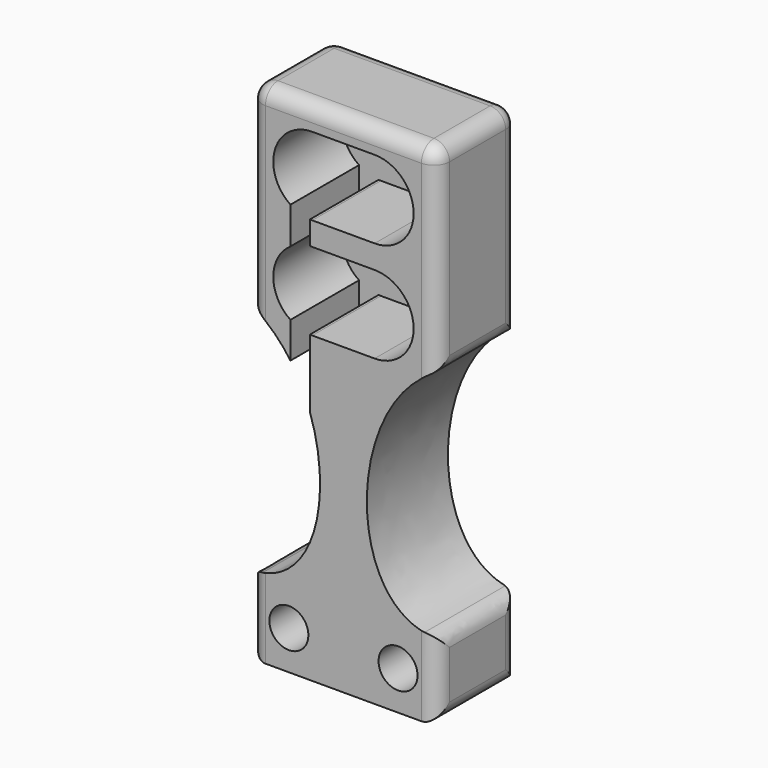
from build123d import *

# Parameters (mm, degrees)
F0_R     = 3.175
F1_DEPTH = 16.51
F2_DEPTH = 2.54
F3_R     = 2.54


# Not quite as in the source:
# - a feature names something its author has since deleted; it is built from what else it names


with BuildPart() as f1:
    # F0 (on Front) → F1 (new body)
    with BuildSketch(Plane.XZ):
        with BuildLine():
            Line((15.24, 10.16), (0, 10.16))
            Line((0, 10.16), (-15.24, 10.16))
            Line((-15.24, 10.16), (-15.24, -21.59))
            add(Edge.make_bspline(
                [(-15.24, -21.59), (-12.5713715272, -23.0241692542), (-10.3700381938, -25.1273333514), (-8.636, -27.620696738)],
                knots=[0, 0, 0, 0, 6.6715711821, 6.6715711821, 6.6715711821, 6.6715711821], degree=3))
            Line((-8.636, -27.620696738), (-8.636, -21.770928055))
            ThreePointArc((-8.636, -21.770928055), (-11.43, -16.51), (-8.636, -11.249071945))
            Line((-8.636, -11.249071945), (-8.636, -5.260928055))
            ThreePointArc((-8.636, -5.260928055), (-11.1516304709, 1.8595169871), (-5.08, 6.35))
            Line((-5.08, 6.35), (5.08, 6.35))
            ThreePointArc((5.08, 6.35), (9.5701280605, 4.4901280605), (11.43, 0))
            ThreePointArc((11.43, 0), (9.5701280605, -4.4901280605), (5.08, -6.35))
            Line((5.08, -6.35), (-5.08, -6.35))
            ThreePointArc((-5.08, -6.35), (-5.2705858603, -6.3471392792), (-5.461, -6.3385596944))
            Line((-5.461, -6.3385596944), (-5.461, -10.1714403056))
            ThreePointArc((-5.461, -10.1714403056), (-5.2705858603, -10.1628607208), (-5.08, -10.16))
            Line((-5.08, -10.16), (5.08, -10.16))
            ThreePointArc((5.08, -10.16), (9.5701280605, -12.0198719395), (11.43, -16.51))
            ThreePointArc((11.43, -16.51), (9.5701280605, -21.0001280605), (5.08, -22.86))
            Line((5.08, -22.86), (-5.08, -22.86))
            ThreePointArc((-5.08, -22.86), (-5.2705858603, -22.8571392792), (-5.461, -22.8485596944))
            Line((-5.461, -22.8485596944), (-5.461, -33.9487214282))
            add(Edge.make_bspline(
                [(-5.461, -33.9487214282), (-1.4642877536, -45.4909328609), (-4.7239544203, -59.7580237479), (-15.24, -59.69)],
                knots=[11.8098860506, 11.8098860506, 11.8098860506, 11.8098860506, 38.1, 38.1, 38.1, 38.1], degree=3))
            Line((-15.24, -59.69), (-15.24, -72.39))
            Line((-15.24, -72.39), (15.24, -72.39))
            Line((15.24, -72.39), (15.24, -59.69))
            add(Edge.make_bspline(
                [(15.24, -21.59), (0, -29.7802519053), (0, -59.7885809647), (15.24, -59.69)],
                knots=[0, 0, 0, 0, 38.1, 38.1, 38.1, 38.1], degree=3))
            Line((15.24, -21.59), (15.24, 10.16))
        make_face()
        with Locations((-8.89, -66.04)):
            Circle(F0_R, mode=Mode.SUBTRACT)
        with Locations((8.89, -66.04)):
            Circle(F0_R, mode=Mode.SUBTRACT)
    extrude(amount=F1_DEPTH)

    # F0 (on Front) → F2 (join)
    with BuildSketch(Plane.XZ):
        with BuildLine():
            ThreePointArc((-5.08, 6.35), (-11.1516304709, 1.8595169871), (-8.636, -5.260928055))
            ThreePointArc((-8.636, -5.260928055), (-7.1209102718, -6.0130845048), (-5.461, -6.3385596944))
            ThreePointArc((-5.461, -6.3385596944), (-5.2705858603, -6.3471392792), (-5.08, -6.35))
            ThreePointArc((-5.08, -6.35), (-2.2401936686, -5.6796126628), (0, -3.81))
            ThreePointArc((0, -3.81), (-1.27, 0), (0, 3.81))
            ThreePointArc((0, 3.81), (-2.2401936686, 5.6796126628), (-5.08, 6.35))
        make_face()
        with BuildLine():
            ThreePointArc((5.08, 6.35), (2.2401936686, 5.6796126628), (0, 3.81))
            ThreePointArc((0, 3.81), (0.9441389426, 2.0080463142), (1.27, 0))
            ThreePointArc((1.27, 0), (0.9441389426, -2.0080463142), (0, -3.81))
            ThreePointArc((0, -3.81), (2.2401936686, -5.6796126628), (5.08, -6.35))
            ThreePointArc((5.08, -6.35), (9.5701280605, -4.4901280605), (11.43, 0))
            ThreePointArc((11.43, 0), (9.5701280605, 4.4901280605), (5.08, 6.35))
        make_face()
        with BuildLine():
            Line((5.08, 6.35), (-5.08, 6.35))
            ThreePointArc((-5.08, 6.35), (-2.2401936686, 5.6796126628), (0, 3.81))
            ThreePointArc((0, 3.81), (2.2401936686, 5.6796126628), (5.08, 6.35))
        make_face()
        with BuildLine():
            ThreePointArc((1.27, 0), (0.9441389426, 2.0080463142), (0, 3.81))
            ThreePointArc((0, 3.81), (-1.27, 0), (0, -3.81))
            ThreePointArc((0, -3.81), (0.9441389426, -2.0080463142), (1.27, 0))
        make_face()
        with BuildLine():
            ThreePointArc((0, -3.81), (-2.2401936686, -5.6796126628), (-5.08, -6.35))
            Line((-5.08, -6.35), (5.08, -6.35))
            ThreePointArc((5.08, -6.35), (2.2401936686, -5.6796126628), (0, -3.81))
        make_face()
        with BuildLine():
            Line((-5.461, -22.5981636269), (-5.461, -22.8485596944))
            ThreePointArc((-5.461, -22.8485596944), (-5.2705858603, -22.8571392792), (-5.08, -22.86))
            ThreePointArc((-5.08, -22.86), (-2.2401936686, -22.1896126628), (0, -20.32))
            ThreePointArc((0, -20.32), (-1.27, -16.51), (0, -12.7))
            ThreePointArc((0, -12.7), (-2.2401936686, -10.8303873372), (-5.08, -10.16))
            ThreePointArc((-5.08, -10.16), (-5.2705858603, -10.1628607208), (-5.461, -10.1714403056))
            Line((-5.461, -10.1714403056), (-5.461, -22.5981636269))
        make_face()
        with BuildLine():
            ThreePointArc((0, -12.7), (-1.27, -16.51), (0, -20.32))
            ThreePointArc((0, -20.32), (0.9441389426, -18.5180463142), (1.27, -16.51))
            ThreePointArc((1.27, -16.51), (0.9441389426, -14.5019536858), (0, -12.7))
        make_face()
        with BuildLine():
            Line((5.08, -10.16), (-5.08, -10.16))
            ThreePointArc((-5.08, -10.16), (-2.2401936686, -10.8303873372), (0, -12.7))
            ThreePointArc((0, -12.7), (2.2401936686, -10.8303873372), (5.08, -10.16))
        make_face()
        with BuildLine():
            ThreePointArc((1.27, -16.51), (0.9441389426, -18.5180463142), (0, -20.32))
            ThreePointArc((0, -20.32), (2.2401936686, -22.1896126628), (5.08, -22.86))
            ThreePointArc((5.08, -22.86), (9.5701280605, -21.0001280605), (11.43, -16.51))
            ThreePointArc((11.43, -16.51), (9.5701280605, -12.0198719395), (5.08, -10.16))
            ThreePointArc((5.08, -10.16), (2.2401936686, -10.8303873372), (0, -12.7))
            ThreePointArc((0, -12.7), (0.9441389426, -14.5019536858), (1.27, -16.51))
        make_face()
        with BuildLine():
            ThreePointArc((0, -20.32), (-2.2401936686, -22.1896126628), (-5.08, -22.86))
            Line((-5.08, -22.86), (5.08, -22.86))
            ThreePointArc((5.08, -22.86), (2.2401936686, -22.1896126628), (0, -20.32))
        make_face()
        with BuildLine():
            Line((-8.636, -21.770928055), (-8.636, -27.620696738))
            add(Edge.make_bspline(
                [(-8.636, -27.620696738), (-7.3004773786, -29.5410369116), (-6.2421440453, -31.6928347959), (-5.461, -33.9487214282)],
                knots=[6.6715711821, 6.6715711821, 6.6715711821, 6.6715711821, 11.8098860506, 11.8098860506, 11.8098860506, 11.8098860506], degree=3))
            Line((-5.461, -33.9487214282), (-5.461, -22.8485596944))
            ThreePointArc((-5.461, -22.8485596944), (-7.1209102718, -22.5230845048), (-8.636, -21.770928055))
        make_face()
        with BuildLine():
            Line((-8.636, -5.260928055), (-8.636, -11.249071945))
            ThreePointArc((-8.636, -11.249071945), (-7.1209102718, -10.4969154952), (-5.461, -10.1714403056))
            Line((-5.461, -10.1714403056), (-5.461, -6.3385596944))
            ThreePointArc((-5.461, -6.3385596944), (-7.1209102718, -6.0130845048), (-8.636, -5.260928055))
        make_face()
        with BuildLine():
            ThreePointArc((-8.636, -11.249071945), (-11.43, -16.51), (-8.636, -21.770928055))
            ThreePointArc((-8.636, -21.770928055), (-7.1209102718, -22.5230845048), (-5.461, -22.8485596944))
            Line((-5.461, -22.8485596944), (-5.461, -22.5981636269))
            Line((-5.461, -22.5981636269), (-5.461, -10.1714403056))
            ThreePointArc((-5.461, -10.1714403056), (-7.1209102718, -10.4969154952), (-8.636, -11.249071945))
        make_face()
    extrude(amount=F2_DEPTH)

    # F3
    f3_edges = [f1.edges().sort_by_distance(p)[0] for p in [
        (15.24, -8.255, 10.16),
        (0, -16.51, 10.16),
        (-15.24, -8.255, 10.16),
        (0, 0, 10.16),
        (15.24, -8.255, -21.59),
        (15.24, 0, -5.715),
        (15.24, -16.51, -5.715),
        (-15.24, -8.255, -21.59),
        (-15.24, 0, -5.715),
        (-15.24, -16.51, -5.715),
        (15.24, -8.255, -72.39),
        (15.24, -8.255, -59.69),
        (15.24, 0, -66.04),
        (15.24, -16.51, -66.04),
        (-15.24, -8.255, -59.69),
        (-15.24, -8.255, -72.39),
        (-15.24, 0, -66.04),
        (-15.24, -16.51, -66.04),
    ]]
    fillet(f3_edges, radius=F3_R)


solid = f1.part
